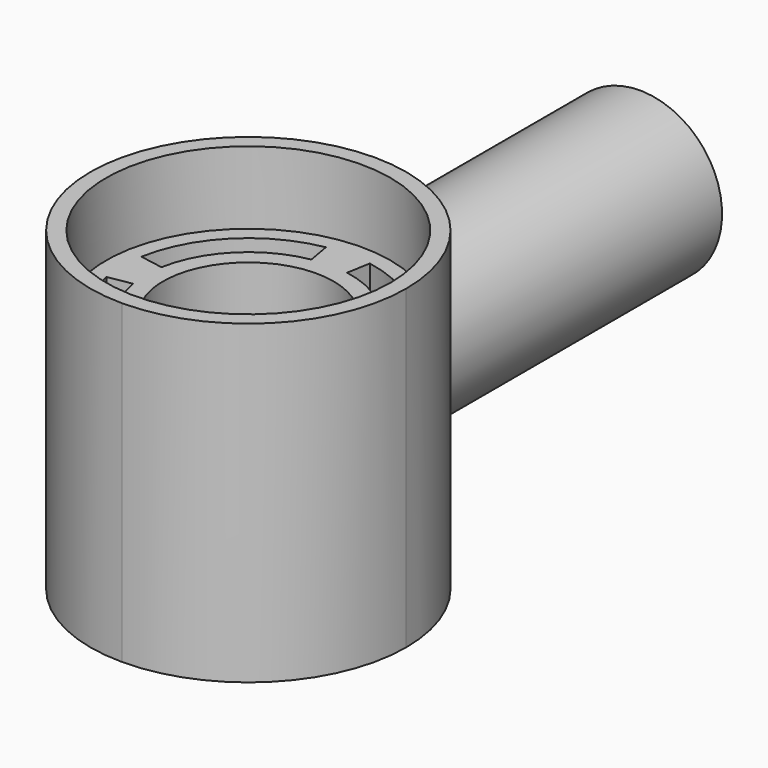
from build123d import *

# Parameters (mm, degrees)
F0_W          = 100
F0_H          = 100
F1_DEPTH      = 50
F2_R          = 27
F3_DEPTH      = 100.001
F4_R          = 45
F5_DEPTH      = 23
F6_R          = 45
F6_R_2        = 27
F7_DEPTH      = 23
F8_R          = 49.99999
F9_R          = 25
F10_DEPTH     = 10
F11_R         = 26
F11_R_2       = 25
F12_DEPTH     = 105
F13_T4_DEPTH  = 100
F13_S5_R      = 26
F13_T6_DEPTH  = 63
F13_T10_DEPTH = 100
F13_S11_R     = 26
F13_T12_DEPTH = 63
F15_DEPTH     = 77.0010001


# Not quite as in the source:
# - a fillet or chamfer that OpenCascade refuses, or shapes differently, is made with other operations: its cross-section is extruded or revolved along the edge and cut away or added
# - a fillet or chamfer is up to 0.001 mm smaller than in the source, because OpenCascade refuses the exact size


with BuildPart() as f1:
    # F0 (on Front) → F1 (new body, symmetric)
    with BuildSketch(Plane.XZ):
        Rectangle(F0_W, F0_H)
    extrude(amount=F1_DEPTH, both=True)

    # F2 (on face) → F3 (cut, through all)
    with BuildSketch(Plane.XY.offset(50)):
        Circle(F2_R)
    extrude(amount=-F3_DEPTH, mode=Mode.SUBTRACT)

    # F4 (on face) → F5 (cut)
    with BuildSketch(Plane.XY.offset(50)):
        Circle(F4_R)
    extrude(amount=-F5_DEPTH, mode=Mode.SUBTRACT)

    # F6 (on face) → F7 (cut)
    with BuildSketch(Plane(origin=(0, 0, -50), x_dir=(1, 0, 0), z_dir=(0, 0, -1))):
        Circle(F6_R)
        Circle(F6_R_2, mode=Mode.SUBTRACT)
    extrude(amount=-F7_DEPTH, mode=Mode.SUBTRACT)

    # F8 (radius 50 in the source; OpenCascade refuses exactly that, so slightly less here)
    f8_edges = [f1.edges().sort_by_distance(p)[0] for p in [
        (50, -50, 0),
        (-50, -50, 0),
    ]]
    fillet(f8_edges, radius=F8_R)

    # F9 (on face) → F10 (cut)
    with BuildSketch(Plane(origin=(0, 50, 0), x_dir=(-1, 0, 0), z_dir=(0, 1, 0))):
        Circle(F9_R)
    extrude(amount=-F10_DEPTH, mode=Mode.SUBTRACT)

    # F11 (on face) → F12 (join)
    with BuildSketch(Plane(origin=(0, 50, 0), x_dir=(-1, 0, 0), z_dir=(0, 1, 0))):
        Circle(F11_R)
        Circle(F11_R_2, mode=Mode.SUBTRACT)
    extrude(amount=F12_DEPTH)

    # F13: fillet of radius 50 on 2 edges, made by hand


with BuildPart() as f13_tool2:
    # F13_s3 → F13_t4 (new body)
    with BuildSketch(Plane.XY.offset(-50)):
        with BuildLine():
            ThreePointArc((50, 0), (35.3553390593, 35.3553390593), (0, 50))
            Line((0, 50), (0, 51))
            Line((0, 51), (51, 51))
            Line((51, 51), (51, 0))
            Line((51, 0), (50, 0))
        make_face()
    extrude(amount=F13_T4_DEPTH)

    # F13_s5 → F13_t6 (cut, symmetric)
    with BuildSketch(Plane.XZ.offset(-25.5)):
        Circle(F13_S5_R)
    extrude(amount=F13_T6_DEPTH, both=True, mode=Mode.SUBTRACT)


with BuildPart() as f1_1:
    add(f1.part)

    # F13_t1: cut F13_tool2
    add(f13_tool2.part, mode=Mode.SUBTRACT)


with BuildPart() as f13_tool8:
    # F13_s9 → F13_t10 (new body)
    with BuildSketch(Plane.XY.offset(50)):
        with BuildLine():
            ThreePointArc((0, 50), (-35.3553390593, 35.3553390593), (-50, 0))
            Line((-50, 0), (-51, 0))
            Line((-51, 0), (-51, 51))
            Line((-51, 51), (0, 51))
            Line((0, 51), (0, 50))
        make_face()
    extrude(amount=-F13_T10_DEPTH)

    # F13_s11 → F13_t12 (cut, symmetric)
    with BuildSketch(Plane.XZ.offset(-25.5)):
        Circle(F13_S11_R)
    extrude(amount=F13_T12_DEPTH, both=True, mode=Mode.SUBTRACT)


with BuildPart() as f1_2:
    add(f1_1.part)

    # F13_t7: cut F13_tool8
    add(f13_tool8.part, mode=Mode.SUBTRACT)

    # F14 (on face) → F15 (cut, through all)
    with BuildSketch(Plane.XY.offset(27)):
        with BuildLine():
            ThreePointArc((-32.0062519729, 5.6435657742), (-22.9809703886, 22.9809703886), (-5.6435657742, 32.0062519729))
            Line((-5.6435657742, 32.0062519729), (-6.9459271067, 39.3923101205))
            ThreePointArc((-6.9459271067, 39.3923101205), (-28.2842712475, 28.2842712475), (-39.3923101205, 6.9459271067))
            Line((-39.3923101205, 6.9459271067), (-32.0062519729, 5.6435657742))
        make_face()
        with BuildLine():
            ThreePointArc((5.6435657742, 32.0062519729), (22.9809703886, 22.9809703886), (32.0062519729, 5.6435657742))
            Line((32.0062519729, 5.6435657742), (39.3923101205, 6.9459271067))
            ThreePointArc((39.3923101205, 6.9459271067), (28.2842712475, 28.2842712475), (6.9459271067, 39.3923101205))
            Line((6.9459271067, 39.3923101205), (5.6435657742, 32.0062519729))
        make_face()
        with BuildLine():
            Line((39.3923101205, -6.9459271067), (32.0062519729, -5.6435657742))
            ThreePointArc((32.0062519729, -5.6435657742), (22.9809703886, -22.9809703886), (5.6435657742, -32.0062519729))
            Line((5.6435657742, -32.0062519729), (6.9459271067, -39.3923101205))
            ThreePointArc((6.9459271067, -39.3923101205), (28.2842712475, -28.2842712475), (39.3923101205, -6.9459271067))
        make_face()
        with BuildLine():
            Line((-6.9459271067, -39.3923101205), (-5.6435657742, -32.0062519729))
            ThreePointArc((-5.6435657742, -32.0062519729), (-22.9809703886, -22.9809703886), (-32.0062519729, -5.6435657742))
            Line((-32.0062519729, -5.6435657742), (-39.3923101205, -6.9459271067))
            ThreePointArc((-39.3923101205, -6.9459271067), (-28.2842712475, -28.2842712475), (-6.9459271067, -39.3923101205))
        make_face()
    extrude(amount=-F15_DEPTH, mode=Mode.SUBTRACT)


solid = f1_2.part
